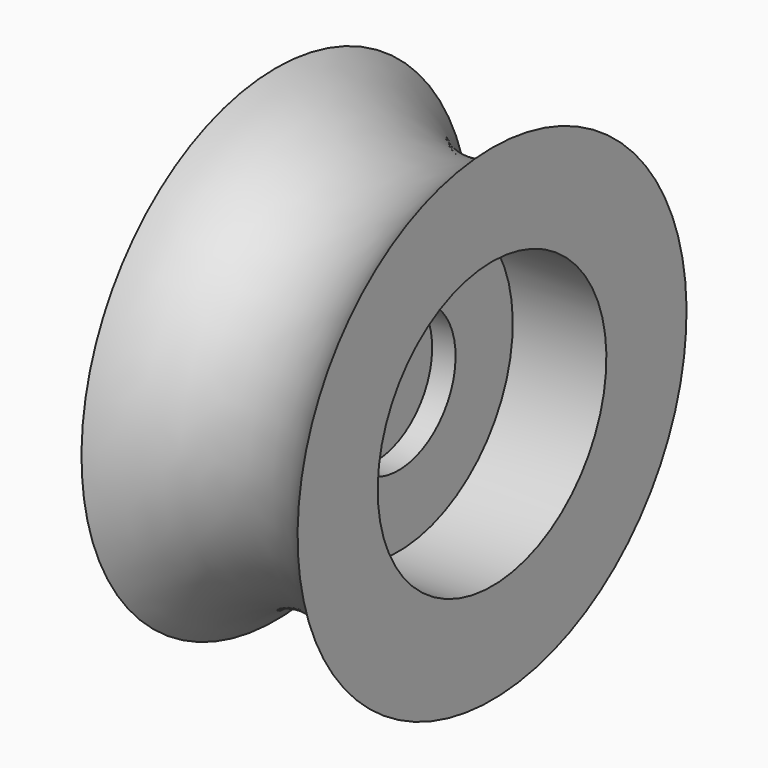
from build123d import *


# Not quite as in the source:
# - a feature names something its author has since deleted; it is built from what else it names


with BuildPart() as f1:
    # F0 (on Front) → F1 (revolve)
    with BuildSketch(Plane.XZ):
        with BuildLine():
            Line((6, 7.9375), (6, 13.5))
            ThreePointArc((6, 13.5), (0, 10.5), (-6, 13.5))
            Line((-6, 13.5), (-6, 7.9375))
            Line((-6, 7.9375), (-0.8, 7.9375))
            Line((-0.8, 7.9375), (-0.8, 0))
            Line((-0.8, 0), (-0.5, 0))
            Line((-0.5, 0), (-0.5, 3.96875))
            Line((-0.5, 3.96875), (0.8, 3.96875))
            Line((0.8, 3.96875), (0.8, 7.9375))
            Line((0.8, 7.9375), (6, 7.9375))
        make_face()
    revolve(axis=Axis((-0.4498892081, 0, 0), (1, 0, 0)))


solid = f1.part
